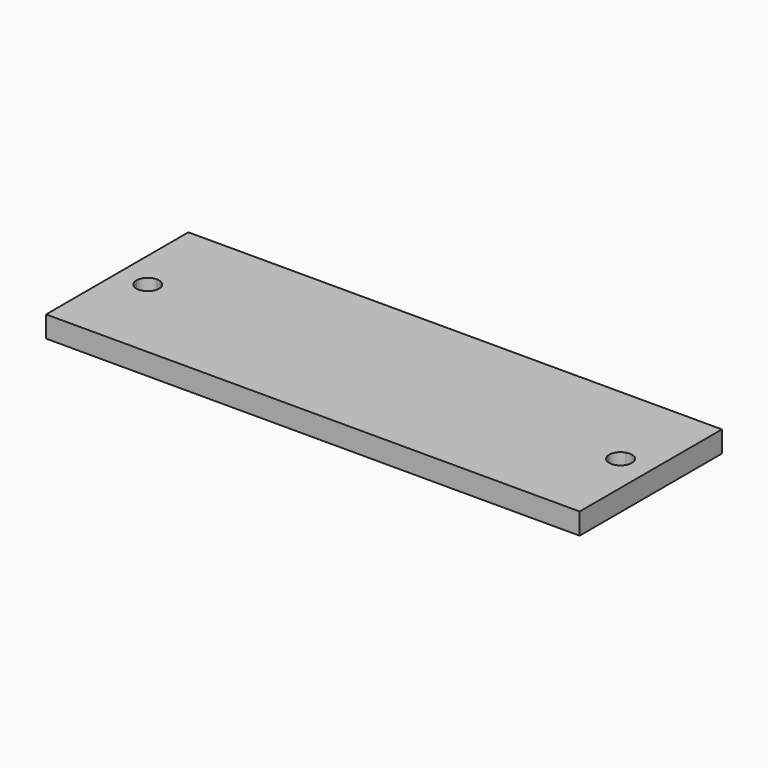
from build123d import *

# Parameters (mm, degrees)
F0_W     = 75
F0_H     = 12.5
F2_DEPTH = 3
F3_DEPTH = 25.4
F1_W     = 30.3805638105
F1_H     = 1.609168168
F1_H_2   = 8.2122374663
F1_H_3   = 1.5025624558
F1_H_4   = 8.1500614509
F4_DEPTH = 0.1
F5_R     = 2.54


# Not quite as in the source:
# - a feature names something its author has since deleted; it is built from what else it names


with BuildPart() as f2:
    # F0 (on Top) → F2 (new body)
    with BuildSketch(Plane.XY):
        with Locations((2.6580473056, -0.5825519562)):
            Rectangle(F0_W, F0_H)
        with Locations((2.6580473056, 11.9174480438)):
            Rectangle(F0_W, F0_H)
    extrude(amount=F2_DEPTH)

    # F1 (on face) → F3 (cut)
    with BuildSketch(Plane.XY):
        with BuildLine():
            ThreePointArc((37.4252376516, 5.6674480438), (37.4269210618, 5.709628552), (37.4274823308, 5.7518389076))
            ThreePointArc((37.4274823308, 5.7518389076), (36.7935957485, 7.0210030812), (35.3981560952, 7.2766162118))
            Line((35.3981560952, 7.2766162118), (35.8816406012, 7.2766162118))
            Line((35.8816406012, 7.2766162118), (35.8816406012, 5.6674480438))
            Line((35.8816406012, 5.6674480438), (37.4252376516, 5.6674480438))
        make_face()
        with BuildLine():
            Line((35.8816406012, 7.2766162118), (35.3981560952, 7.2766162118))
            ThreePointArc((35.3981560952, 7.2766162118), (34.5459110587, 6.6713691097), (34.25472701, 5.6674480438))
            Line((34.25472701, 5.6674480438), (35.8816406012, 5.6674480438))
            Line((35.8816406012, 5.6674480438), (35.8816406012, 7.2766162118))
        make_face()
        with BuildLine():
            ThreePointArc((35.8816406012, 4.164885588), (36.9472923333, 4.6142885534), (37.4252376516, 5.6674480438))
            Line((37.4252376516, 5.6674480438), (35.8816406012, 5.6674480438))
            Line((35.8816406012, 5.6674480438), (35.8816406012, 4.164885588))
        make_face()
        with BuildLine():
            Line((35.8816406012, 5.6674480438), (34.25472701, 5.6674480438))
            ThreePointArc((34.25472701, 5.6674480438), (34.7326723283, 4.6142885534), (35.7983240604, 4.164885588))
            Line((35.7983240604, 4.164885588), (35.8816406012, 4.164885588))
            Line((35.8816406012, 4.164885588), (35.8816406012, 5.6674480438))
        make_face()
        with BuildLine():
            Line((-30.5555813976, 5.6674480438), (-30.5555813976, 7.2766162118))
            ThreePointArc((-30.5555813976, 7.2766162118), (-31.6926900402, 6.8077826631), (-32.1536216159, 5.6674480438))
            Line((-32.1536216159, 5.6674480438), (-30.5555813976, 5.6674480438))
        make_face()
        with BuildLine():
            ThreePointArc((-28.9787699914, 5.6891521952), (-29.4399653273, 6.8078988393), (-30.5555813976, 7.2766162118))
            Line((-30.5555813976, 7.2766162118), (-30.5555813976, 5.6674480438))
            Line((-30.5555813976, 5.6674480438), (-28.9789183669, 5.6674480438))
            ThreePointArc((-28.9789183669, 5.6674480438), (-28.9788070858, 5.678299866), (-28.9787699914, 5.6891521952))
        make_face()
        with BuildLine():
            ThreePointArc((-30.1226850953, 4.164885588), (-29.303099666, 4.7276133355), (-28.9789183669, 5.6674480438))
            Line((-28.9789183669, 5.6674480438), (-30.5555813976, 5.6674480438))
            Line((-30.5555813976, 5.6674480438), (-30.5555813976, 4.164885588))
            Line((-30.5555813976, 4.164885588), (-30.1226850953, 4.164885588))
        make_face()
        with BuildLine():
            Line((-30.5555813976, 5.6674480438), (-32.1536216159, 5.6674480438))
            ThreePointArc((-32.1536216159, 5.6674480438), (-31.5104490346, 4.4129538625), (-30.1226850953, 4.164885588))
            Line((-30.1226850953, 4.164885588), (-30.5555813976, 4.164885588))
            Line((-30.5555813976, 4.164885588), (-30.5555813976, 5.6674480438))
        make_face()
    extrude(amount=F3_DEPTH, mode=Mode.SUBTRACT)

    # F1 (on face) → F4 (cut)
    with BuildSketch(Plane.XY):
        with BuildLine():
            ThreePointArc((34.25472701, 5.6674480438), (34.5459110587, 6.6713691097), (35.3981560952, 7.2766162118))
            Line((35.3981560952, 7.2766162118), (15.1902819052, 7.2766162118))
            Line((15.1902819052, 7.2766162118), (15.1902819052, 5.6674480438))
            Line((15.1902819052, 5.6674480438), (34.25472701, 5.6674480438))
        make_face()
        with BuildLine():
            ThreePointArc((35.7983240604, 4.164885588), (34.7326723283, 4.6142885534), (34.25472701, 5.6674480438))
            Line((34.25472701, 5.6674480438), (15.1902819052, 5.6674480438))
            Line((15.1902819052, 5.6674480438), (15.1902819052, 4.164885588))
            Line((15.1902819052, 4.164885588), (35.7983240604, 4.164885588))
        make_face()
        with Locations((0, 6.4720321278)):
            Rectangle(F1_W, F1_H)
        with Locations((0, 11.382734945)):
            Rectangle(F1_W, F1_H_2)
        with Locations((0, 4.9161668159)):
            Rectangle(F1_W, F1_H_3)
        with BuildLine():
            Line((-15.1902819052, 5.6674480438), (-15.1902819052, 7.2766162118))
            Line((-15.1902819052, 7.2766162118), (-30.5555813976, 7.2766162118))
            ThreePointArc((-30.5555813976, 7.2766162118), (-29.4399653273, 6.8078988393), (-28.9787699914, 5.6891521952))
            ThreePointArc((-28.9787699914, 5.6891521952), (-28.9788070858, 5.678299866), (-28.9789183669, 5.6674480438))
            Line((-28.9789183669, 5.6674480438), (-15.1902819052, 5.6674480438))
        make_face()
        with Locations((0, 0.0898548626)):
            Rectangle(F1_W, F1_H_4)
        with BuildLine():
            Line((-15.1902819052, 4.164885588), (-15.1902819052, 5.6674480438))
            Line((-15.1902819052, 5.6674480438), (-28.9789183669, 5.6674480438))
            ThreePointArc((-28.9789183669, 5.6674480438), (-29.303099666, 4.7276133355), (-30.1226850953, 4.164885588))
            Line((-30.1226850953, 4.164885588), (-15.1902819052, 4.164885588))
        make_face()
    extrude(amount=F4_DEPTH, mode=Mode.SUBTRACT)

    # F5
    f5_edges = [f2.edges().sort_by_distance(p)[0] for p in [
        (-15.190282, 4.164886, 0.05),
        (-15.190282, 7.276616, 0.05),
        (15.190282, 4.164886, 0.05),
        (15.190282, 7.276616, 0.05),
    ]]
    fillet(f5_edges, radius=F5_R)


solid = f2.part
